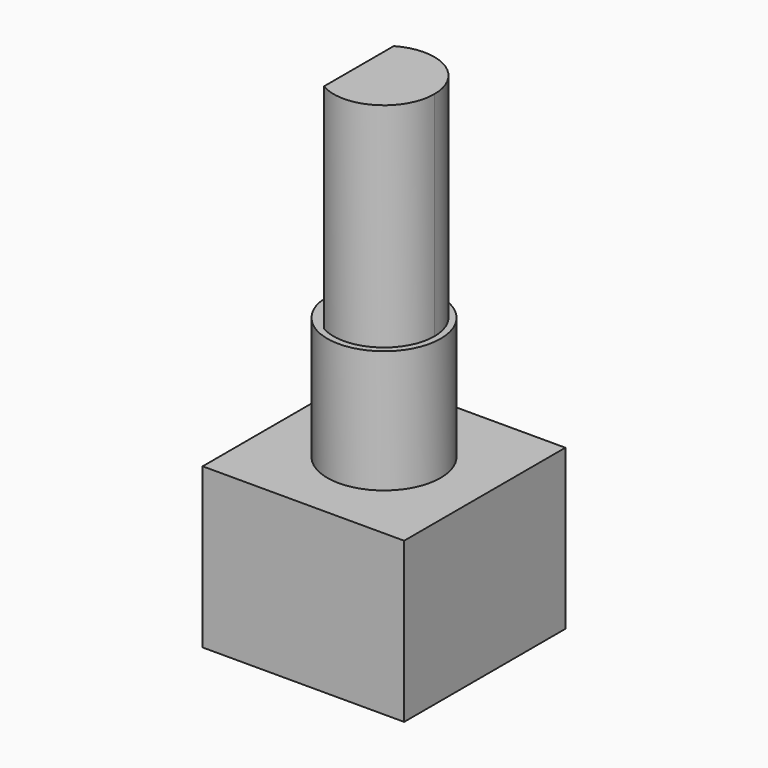
from build123d import *

# Parameters (mm, degrees)
F0_W     = 12
F0_H     = 12
F0_R     = 3.375
F1_DEPTH = 9.5
F2_DEPTH = 7.3
F3_DEPTH = 20


with BuildPart() as f1:
    # F0 (on Top) → F1 (new body)
    with BuildSketch(Plane.XY):
        Rectangle(F0_W, F0_H)
        Circle(F0_R, mode=Mode.SUBTRACT)
        Circle(F0_R)
        with BuildLine():
            ThreePointArc((-1.5, 2.5980762114), (1.5, 2.5980762114), (3, 0))
            ThreePointArc((3, 0), (1.5, -2.5980762114), (-1.5, -2.5980762114))
            ThreePointArc((-1.5, -2.5980762114), (-3, 0), (-1.5, 2.5980762114))
        make_face(mode=Mode.SUBTRACT)
        with BuildLine():
            ThreePointArc((-1.5, -2.5980762114), (1.5, -2.5980762114), (3, 0))
            ThreePointArc((3, 0), (1.5, 2.5980762114), (-1.5, 2.5980762114))
            Line((-1.5, 2.5980762114), (-1.5, -2.5980762114))
        make_face()
        with BuildLine():
            Line((-1.5, -2.5980762114), (-1.5, 2.5980762114))
            ThreePointArc((-1.5, 2.5980762114), (-3, 0), (-1.5, -2.5980762114))
        make_face()
    extrude(amount=-F1_DEPTH)

    # F0 (on Top) → F2 (join)
    with BuildSketch(Plane.XY):
        Circle(F0_R)
        with BuildLine():
            ThreePointArc((-1.5, 2.5980762114), (1.5, 2.5980762114), (3, 0))
            ThreePointArc((3, 0), (1.5, -2.5980762114), (-1.5, -2.5980762114))
            ThreePointArc((-1.5, -2.5980762114), (-3, 0), (-1.5, 2.5980762114))
        make_face(mode=Mode.SUBTRACT)
        with BuildLine():
            ThreePointArc((-1.5, -2.5980762114), (1.5, -2.5980762114), (3, 0))
            ThreePointArc((3, 0), (1.5, 2.5980762114), (-1.5, 2.5980762114))
            Line((-1.5, 2.5980762114), (-1.5, -2.5980762114))
        make_face()
        with BuildLine():
            Line((-1.5, -2.5980762114), (-1.5, 2.5980762114))
            ThreePointArc((-1.5, 2.5980762114), (-3, 0), (-1.5, -2.5980762114))
        make_face()
    extrude(amount=F2_DEPTH)

    # F0 (on Top) → F3 (join)
    with BuildSketch(Plane.XY):
        with BuildLine():
            ThreePointArc((-1.5, -2.5980762114), (1.5, -2.5980762114), (3, 0))
            ThreePointArc((3, 0), (1.5, 2.5980762114), (-1.5, 2.5980762114))
            Line((-1.5, 2.5980762114), (-1.5, -2.5980762114))
        make_face()
    extrude(amount=F3_DEPTH)


solid = f1.part
